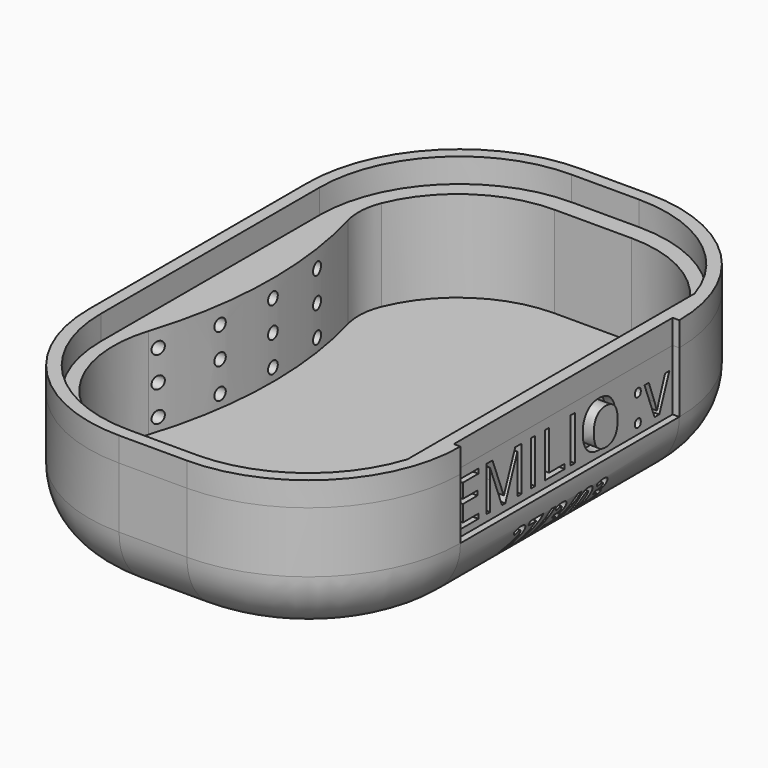
from build123d import *

# Parameters (mm, degrees)
F1_DEPTH       = 15
F3_W           = 61.16227
F3_H           = 95
F4_DEPTH       = 20
F6_R           = 25
F7_R           = 10
F8_W           = 45
F8_H           = 10
F8_W_2         = 0.8474005249
F8_H_2         = 7.2914745727
F9_DEPTH       = 1.1
F8_TEXT_SIZE   = 10.2134903185
F8_TEXT_SIZE_2 = 5.5456329448
F10_DEPTH      = 2.8
F11_R          = 1
F12_DEPTH      = 25
F14_DEPTH      = 4


# Not quite as in the source:
# - Text() gives the source's letters only with a copy of the font that has no kerning and outlines rounded to 1/6400 em; it was checked with that copy


with BuildPart() as f1:
    # F0 (on Top) → F1 (new body)
    with BuildSketch(Plane.XY):
        with BuildLine():
            Line((32.3356321475, 85), (19.6643678525, 85))
            ThreePointArc((19.6643678525, 85), (8.4955603594, 81.5908932605), (1.1343185559, 72.5257739181))
            ThreePointArc((1.1343185559, 72.5257739181), (0.4158743323, 69.3376471556), (0.7636959679, 66.0881341973))
            ThreePointArc((0.7636959679, 66.0881341973), (3.3014151062, 46.0288759253), (0, 26.0810810811))
            ThreePointArc((0, 26.0810810811), (2.9034575232, 8.2021531969), (19.0530956247, 0))
            Line((19.0530956247, 0), (32.9469043753, 0))
            ThreePointArc((32.9469043753, 0), (49.0965424768, 8.2021531969), (52, 26.0810810811))
            ThreePointArc((52, 26.0810810811), (48.6985848938, 46.0288759253), (51.2363040321, 66.0881341973))
            ThreePointArc((51.2363040321, 66.0881341973), (51.5841256677, 69.3376471556), (50.8656814441, 72.5257739181))
            ThreePointArc((50.8656814441, 72.5257739181), (43.5044396406, 81.5908932605), (32.3356321475, 85))
        make_face()
    extrude(amount=-F1_DEPTH)


with BuildPart() as f4:
    # F3 (on offset) → F4 (new body)
    with BuildSketch(Plane.XY.offset(-20)):
        with Locations((25.581135, 42.5)):
            Rectangle(F3_W, F3_H)
    extrude(amount=F4_DEPTH)

    # F5: cut F1
    add(f1.part, mode=Mode.SUBTRACT)

    # F6
    f6_edges = [f4.edges().sort_by_distance(p)[0] for p in [
        (-5, 90, -10),
        (-5, -5, -10),
        (56.16227, -5, -10),
        (56.16227, 90, -10),
    ]]
    fillet(f6_edges, radius=F6_R)

    # F7
    f7_edges = [f4.edges().sort_by_distance(p)[0] for p in [
        (56.16227, 42.5, -20),
        (48.83994, 2.32233, -20),
        (48.83994, 82.67767, -20),
        (25.581135, -5, -20),
        (25.581135, 90, -20),
        (2.32233, 2.32233, -20),
        (2.32233, 82.67767, -20),
        (-5, 42.5, -20),
    ]]
    fillet(f7_edges, radius=F7_R)

    # F8 (on face) → F9 (cut)
    with BuildSketch(Plane.YZ.offset(56.16227)):
        with Locations((42.5, -5)):
            Rectangle(F8_W, F8_H)
        Polygon((25.0668487127, -8.13027296), (25.0668487127, -8.8883054445), (21.0021987375, -8.8883054445), (21.0021987375, -1.5968308719), (25.0668487127, -1.5968308719), (25.0668487127, -2.3500757829), (21.8495992624, -2.3500757829), (21.8495992624, -4.6991785561), (24.8721540535, -4.6991785561), (24.8721540535, -5.4476358935), (21.8495992624, -5.4476358935), (21.8495992624, -8.13027296), align=None, mode=Mode.SUBTRACT)
        with BuildLine():
            Line((30.5917086318, -8.8883054445), (29.9086814668, -8.8883054445))
            Line((29.9086814668, -8.8883054445), (27.4351017803, -2.4250811024))
            Line((27.4351017803, -2.4250811024), (27.3952053337, -2.4250811024))
            add(Edge.make_bspline(
                [(27.3952053337, -2.4250811024), (27.4654230797, -3.1926887341), (27.4654230797, -4.2507424968)],
                knots=[0, 0, 0, 1, 1, 1], degree=2))
            Line((27.4654230797, -4.2507424968), (27.4654230797, -8.8883054445))
            Line((27.4654230797, -8.8883054445), (26.6818568693, -8.8883054445))
            Line((26.6818568693, -8.8883054445), (26.6818568693, -1.5968308719))
            Line((26.6818568693, -1.5968308719), (27.9585431591, -1.5968308719))
            Line((27.9585431591, -1.5968308719), (30.2677494858, -7.6116191547))
            Line((30.2677494858, -7.6116191547), (30.3076459323, -7.6116191547))
            Line((30.3076459323, -7.6116191547), (32.6360025534, -1.5968308719))
            Line((32.6360025534, -1.5968308719), (33.903113696, -1.5968308719))
            Line((33.903113696, -1.5968308719), (33.903113696, -8.8883054445))
            Line((33.903113696, -8.8883054445), (33.0557131711, -8.8883054445))
            Line((33.0557131711, -8.8883054445), (33.0557131711, -4.1900998981))
            add(Edge.make_bspline(
                [(33.0557131711, -4.1900998981), (33.0557131711, -3.3825958197), (33.1259309171, -2.4346562496)],
                knots=[0, 0, 0, 1, 1, 1], degree=2))
            Line((33.1259309171, -2.4346562496), (33.0860344705, -2.4346562496))
            Line((33.0860344705, -2.4346562496), (30.5917086318, -8.8883054445))
        make_face(mode=Mode.SUBTRACT)
        with Locations((36.3264238598, -5.2425681582)):
            Rectangle(F8_W_2, F8_H_2, mode=Mode.SUBTRACT)
        Polygon((42.8143839989, -8.8883054445), (38.7497340237, -8.8883054445), (38.7497340237, -1.5968308719), (39.5971345485, -1.5968308719), (39.5971345485, -8.1206978128), (42.8143839989, -8.1206978128), align=None, mode=Mode.SUBTRACT)
        with Locations((44.4748741045, -5.2425681582)):
            Rectangle(F8_W_2, F8_H_2, mode=Mode.SUBTRACT)
        with BuildLine():
            add(Edge.make_bspline(
                [(52.3448471523, -2.4793402697), (53.2273565501, -3.4767514336), (53.2273565501, -5.2321950821)],
                knots=[0, 0, 0, 1, 1, 1], degree=2))
            add(Edge.make_bspline(
                [(53.2273565501, -5.2321950821), (53.2273565501, -6.982851157), (52.3416554366, -7.9858478234)],
                knots=[0, 0, 0, 1, 1, 1], degree=2))
            add(Edge.make_bspline(
                [(52.3416554366, -7.9858478234), (51.455954323, -8.9888444899), (49.880842613, -8.9888444899)],
                knots=[0, 0, 0, 1, 1, 1], degree=2))
            add(Edge.make_bspline(
                [(49.880842613, -8.9888444899), (48.2706220299, -8.9888444899), (47.3952939925, -8.0034022599)],
                knots=[0, 0, 0, 1, 1, 1], degree=2))
            add(Edge.make_bspline(
                [(47.3952939925, -8.0034022599), (46.519965955, -7.01796003), (46.519965955, -5.2226199349)],
                knots=[0, 0, 0, 1, 1, 1], degree=2))
            add(Edge.make_bspline(
                [(46.519965955, -5.2226199349), (46.519965955, -3.4416425607), (47.3976877793, -2.4617858332)],
                knots=[0, 0, 0, 1, 1, 1], degree=2))
            add(Edge.make_bspline(
                [(47.3976877793, -2.4617858332), (48.2754096035, -1.4819291058), (49.8904177601, -1.4819291058)],
                knots=[0, 0, 0, 1, 1, 1], degree=2))
            add(Edge.make_bspline(
                [(49.8904177601, -1.4819291058), (51.4623377545, -1.4819291058), (52.3448471523, -2.4793402697)],
                knots=[0, 0, 0, 1, 1, 1], degree=2))
        make_face(mode=Mode.SUBTRACT)
        with BuildLine():
            add(Edge.make_bspline(
                [(57.4284523725, -8.8763365106), (57.2616852259, -8.7191445111), (57.2616852259, -8.3600764921)],
                knots=[0, 0, 0, 1, 1, 1], degree=2))
            add(Edge.make_bspline(
                [(57.2616852259, -8.3600764921), (57.2616852259, -8.0249463411), (57.4140896517, -7.8533916209)],
                knots=[0, 0, 0, 1, 1, 1], degree=2))
            add(Edge.make_bspline(
                [(57.4140896517, -7.8533916209), (57.5664940776, -7.6818369007), (57.8505567771, -7.6818369007)],
                knots=[0, 0, 0, 1, 1, 1], degree=2))
            add(Edge.make_bspline(
                [(57.8505567771, -7.6818369007), (58.1394070501, -7.6818369007), (58.3013866232, -7.8533916209)],
                knots=[0, 0, 0, 1, 1, 1], degree=2))
            add(Edge.make_bspline(
                [(58.3013866232, -7.8533916209), (58.4633661962, -8.0249463411), (58.4633661962, -8.3600764921)],
                knots=[0, 0, 0, 1, 1, 1], degree=2))
            add(Edge.make_bspline(
                [(58.4633661962, -8.3600764921), (58.4633661962, -8.6840356382), (58.2989928364, -8.8587820741)],
                knots=[0, 0, 0, 1, 1, 1], degree=2))
            add(Edge.make_bspline(
                [(58.2989928364, -8.8587820741), (58.1346194766, -9.03352851), (57.8505567771, -9.03352851)],
                knots=[0, 0, 0, 1, 1, 1], degree=2))
            add(Edge.make_bspline(
                [(57.8505567771, -9.03352851), (57.5952195191, -9.03352851), (57.4284523725, -8.8763365106)],
                knots=[0, 0, 0, 1, 1, 1], degree=2))
        make_face(mode=Mode.SUBTRACT)
        with BuildLine():
            Line((62.2631037662, -8.8883054445), (61.2960139017, -8.8883054445))
            Line((61.2960139017, -8.8883054445), (59.2213986808, -3.4224922663))
            Line((59.2213986808, -3.4224922663), (60.1086956522, -3.4224922663))
            Line((60.1086956522, -3.4224922663), (61.2864387545, -6.6636795846))
            add(Edge.make_bspline(
                [(61.2864387545, -6.6636795846), (61.6854032201, -7.8015262403), (61.755620966, -8.1398481071)],
                knots=[0, 0, 0, 1, 1, 1], degree=2))
            Line((61.755620966, -8.1398481071), (61.7955174126, -8.1398481071))
            add(Edge.make_bspline(
                [(61.7955174126, -8.1398481071), (61.8497765799, -7.8765315599), (62.1418185687, -7.0458875426)],
                knots=[0, 0, 0, 1, 1, 1], degree=2))
            add(Edge.make_bspline(
                [(62.1418185687, -7.0458875426), (62.4338605575, -6.2152435253), (63.4504220157, -3.4224922663)],
                knots=[0, 0, 0, 1, 1, 1], degree=2))
            Line((63.4504220157, -3.4224922663), (64.3377189872, -3.4224922663))
            Line((64.3377189872, -3.4224922663), (62.2631037662, -8.8883054445))
        make_face(mode=Mode.SUBTRACT)
        with BuildLine():
            add(Edge.make_bspline(
                [(57.4284523725, -4.4717688107), (57.2616852259, -4.3145768113), (57.2616852259, -3.9555087923)],
                knots=[0, 0, 0, 1, 1, 1], degree=2))
            add(Edge.make_bspline(
                [(57.2616852259, -3.9555087923), (57.2616852259, -3.2820567744), (57.8505567771, -3.2820567744)],
                knots=[0, 0, 0, 1, 1, 1], degree=2))
            add(Edge.make_bspline(
                [(57.8505567771, -3.2820567744), (58.4633661962, -3.2820567744), (58.4633661962, -3.9555087923)],
                knots=[0, 0, 0, 1, 1, 1], degree=2))
            add(Edge.make_bspline(
                [(58.4633661962, -3.9555087923), (58.4633661962, -4.2794679383), (58.2989928364, -4.4542143743)],
                knots=[0, 0, 0, 1, 1, 1], degree=2))
            add(Edge.make_bspline(
                [(58.2989928364, -4.4542143743), (58.1346194766, -4.6289608102), (57.8505567771, -4.6289608102)],
                knots=[0, 0, 0, 1, 1, 1], degree=2))
            add(Edge.make_bspline(
                [(57.8505567771, -4.6289608102), (57.5952195191, -4.6289608102), (57.4284523725, -4.4717688107)],
                knots=[0, 0, 0, 1, 1, 1], degree=2))
        make_face(mode=Mode.SUBTRACT)
    extrude(amount=-F9_DEPTH, mode=Mode.SUBTRACT)

    # F8 (on face) → F10 (cut)
    with BuildSketch(Plane.YZ.offset(56.16227)):
        with Locations((20, -8.8883054445)):
            Text('EMILIO :v', F8_TEXT_SIZE, font='Open Sans', text_align=(TextAlign.LEFT, TextAlign.BOTTOM))
        with Locations((31.2811714903, -16.9928557202)):
            Text('27/3/03', F8_TEXT_SIZE_2, font='Open Sans', font_style=FontStyle.BOLDITALIC, text_align=(TextAlign.LEFT, TextAlign.BOTTOM))
    extrude(amount=-F10_DEPTH, mode=Mode.SUBTRACT)

    # F11 (on face) → F12 (cut)
    with BuildSketch(Plane(origin=(-5, 0, 0), x_dir=(0, -1, 0), z_dir=(-1, 0, 0))):
        with Locations((-57.5, -12.8899160542)):
            Circle(F11_R)
        with Locations((-57.5, -7.8899160542)):
            Circle(F11_R)
        with Locations((-57.5, -2.8899160542)):
            Circle(F11_R)
        with Locations((-47.5, -12.8899160542)):
            Circle(F11_R)
        with Locations((-47.5, -7.8899160542)):
            Circle(F11_R)
        with Locations((-47.5, -2.8899160542)):
            Circle(F11_R)
        with Locations((-37.5, -12.8899160542)):
            Circle(F11_R)
        with Locations((-37.5, -7.8899160542)):
            Circle(F11_R)
        with Locations((-37.5, -2.8899160542)):
            Circle(F11_R)
        with Locations((-27.5, -12.8899160542)):
            Circle(F11_R)
        with Locations((-27.5, -7.8899160542)):
            Circle(F11_R)
        with Locations((-27.5, -2.8899160542)):
            Circle(F11_R)
    extrude(amount=-F12_DEPTH, mode=Mode.SUBTRACT)

    # F13 (on face) → F14 (join)
    with BuildSketch(Plane.XY):
        with BuildLine():
            Line((20, -5), (31.16227, -5))
            ThreePointArc((31.16227, -5), (48.8399395297, 2.3223304703), (56.16227, 20))
            Line((56.16227, 20), (55.06227, 20))
            Line((55.06227, 20), (55.06227, 65))
            Line((55.06227, 65), (56.16227, 65))
            ThreePointArc((56.16227, 65), (48.8399395297, 82.6776695297), (31.16227, 90))
            Line((31.16227, 90), (20, 90))
            ThreePointArc((20, 90), (2.3223304703, 82.6776695297), (-5, 65))
            Line((-5, 65), (-5, 20))
            ThreePointArc((-5, 20), (2.3223304703, 2.3223304703), (20, -5))
        make_face()
        with BuildLine():
            ThreePointArc((53.06227, 12.9721980677), (44.7151397248, 1.4172197392), (31.16227, -3))
            Line((31.16227, -3), (20, -3))
            ThreePointArc((20, -3), (3.7365440327, 3.7365440327), (-3, 20))
            Line((-3, 20), (-3, 65))
            ThreePointArc((-3, 65), (3.7365440327, 81.2634559673), (20, 88))
            Line((20, 88), (31.16227, 88))
            ThreePointArc((31.16227, 88), (44.7151397248, 83.5827802608), (53.06227, 72.0278019323))
            Line((53.06227, 72.0278019323), (53.06227, 12.9721980677))
        make_face(mode=Mode.SUBTRACT)
    extrude(amount=F14_DEPTH)


solid = f4.part
